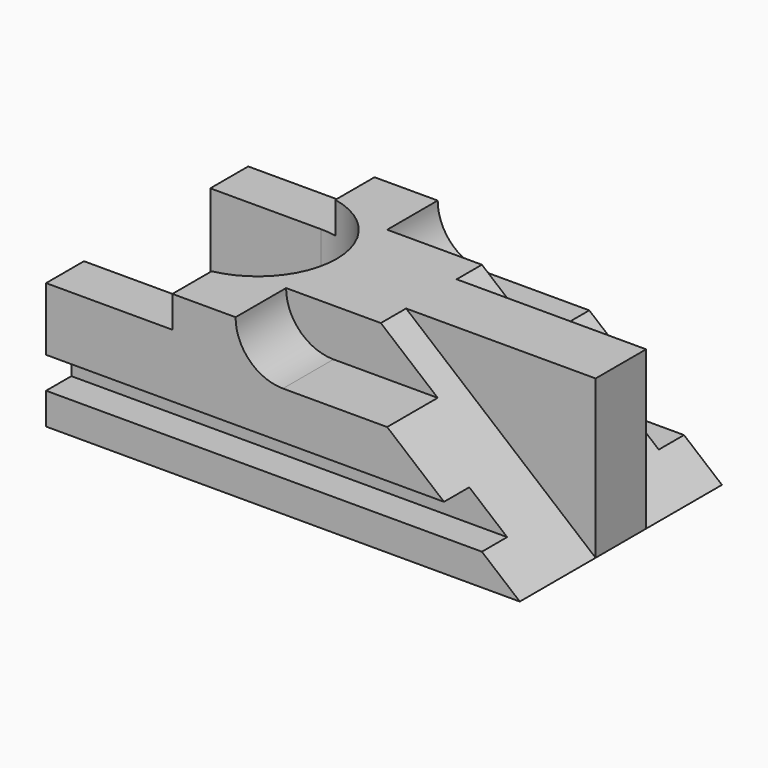
from build123d import *

# Parameters (mm, degrees)
F1_DEPTH = 50
F2_W     = 40
F2_H     = 10
F3_DEPTH = 30
F4_DEPTH = 10
F5_DEPTH = 20


# Not quite as in the source:
# - a pattern or mirror of a feature is missing from the dataset's text; its kind, count and spacing are read off the source's solid


with BuildPart() as f1:
    # F0 (on Top) → F1 (new body)
    with BuildSketch(Plane.XY):
        with BuildLine():
            Line((-35, -25), (-35, -40))
            Line((-35, -40), (115, -40))
            Line((115, -40), (115, 40))
            Line((115, 40), (-35, 40))
            Line((-35, 40), (-35, 25))
            Line((-35, 25), (0, 25))
            ThreePointArc((0, 25), (25, 0), (0, -25))
            Line((0, -25), (-35, -25))
        make_face()
    extrude(amount=F1_DEPTH)

    # F2 (on face) → F3 (cut)
    with BuildSketch(Plane.XZ.offset(40)):
        with Locations((-15, 45)):
            Rectangle(F2_W, F2_H)
        Polygon((115, 50), (55, 50), (73, 35), (91, 20), (103, 10), (115, 0), align=None)
    f3 = extrude(amount=-F3_DEPTH, mode=Mode.SUBTRACT)

    # F3_copies: F3 across plane
    add(f3.mirror(Plane.ZX), mode=Mode.SUBTRACT)

    # F2 (on face) → F4 (cut)
    with BuildSketch(Plane.XZ.offset(40)):
        Polygon((91, 20), (-35, 20), (-35, 10), (103, 10), align=None)
    f4 = extrude(amount=-F4_DEPTH, mode=Mode.SUBTRACT)

    # F4_copies: F4 across plane
    add(f4.mirror(Plane.ZX), mode=Mode.SUBTRACT)

    # F2 (on face) → F5 (cut)
    with BuildSketch(Plane.XZ.offset(40)):
        with BuildLine():
            Line((55, 50), (25, 50))
            ThreePointArc((25, 50), (29.3933982822, 39.3933982822), (40, 35))
            Line((40, 35), (73, 35))
            Line((73, 35), (55, 50))
        make_face()
    f5 = extrude(amount=-F5_DEPTH, mode=Mode.SUBTRACT)

    # F5_copies: F5 across plane
    add(f5.mirror(Plane.ZX), mode=Mode.SUBTRACT)


solid = f1.part
